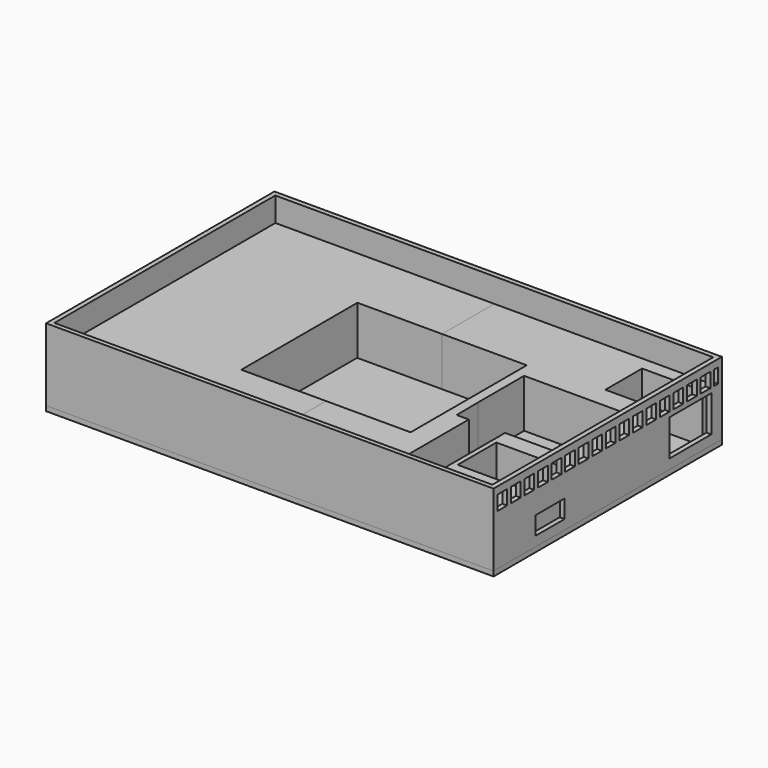
from build123d import *

# Parameters (mm, degrees)
F1_DEPTH = 2
F0_W     = 41
F0_H     = 23.8580039246
F0_W_2   = 35
F0_H_2   = 30
F0_W_3   = 14.5
F0_H_3   = 19
F0_W_4   = 10.5
F3_DEPTH = 22
F4_DEPTH = 30
F5_W     = 29.3693448901
F5_H     = 20
F6_DEPTH = 22
F7_W     = 5
F7_H     = 6
F7_W_2   = 2
F7_W_3   = 15
F7_H_2   = 7.5
F7_W_4   = 21.5
F7_H_3   = 15
F8_DEPTH = 2


with BuildPart() as f1:
    # F0 (on Top) → F1 (new body)
    with BuildSketch(Plane.XY):
        Polygon((29.8828537283, 118), (-155.1171462717, 118), (-155.1171462717, 0), (29.8828537283, 0), (29.8828537283, 47.8673752217), align=None)
        Polygon((27.8828537283, 108.5818558931), (27.8828537283, 47.8439224922), (27.8828537283, 9.4181441069), (27.8828537283, 2), (27.8251939824, 2), (27.8251939824, 1.8636477081), (-62.6748060176, 1.8636477081), (-153.1748060176, 1.8636477081), (-153.1748060176, 58.8636477081), (-153.1748060176, 115.8636477081), (-153.1171462717, 115.8636477081), (-153.1171462717, 116), (27.8828537283, 116), align=None, mode=Mode.SUBTRACT)
    extrude(amount=F1_DEPTH)


with BuildPart() as f1b:
    # F0 (on Top) → F1, piece 2 (new body)
    with BuildSketch(Plane.XY):
        Polygon((27.8251939824, 20.7216516327), (27.8251939824, 40.7216516327), (-1.5441509077, 40.7216516327), (-1.5441509077, 30.7216516327), (-1.5441509077, 20.7216516327), align=None)
    extrude(amount=F1_DEPTH)


with BuildPart() as f1c:
    # F0 (on Top) → F1, piece 3 (new body)
    with BuildSketch(Plane.XY):
        Polygon((-1.5441509077, 47.7216516327), (17.4558490923, 47.7216516327), (17.3251939824, 58.8636477081), (-23.6748060176, 58.8636477081), (-23.5441509077, 47.7216516327), (-18.5441509077, 47.7216516327), (-18.5441509077, 13.7216516327), (-3.5441509077, 13.7216516327), (-3.5441509077, 47.7216516327), align=None)
        with Locations((-3.1748060176, 70.7926496704)):
            Rectangle(F0_W, F0_H)
    extrude(amount=F1_DEPTH)


with BuildPart() as f1d:
    # F0 (on Top) → F1, piece 4 (new body)
    with BuildSketch(Plane.XY):
        with Locations((-45.1748060176, 73.8636477081)):
            Rectangle(F0_W_2, F0_H_2)
        with Locations((-80.1748060176, 73.8636477081)):
            Rectangle(F0_W_2, F0_H_2)
        with Locations((-80.1748060176, 43.8636477081)):
            Rectangle(F0_W_2, F0_H_2)
        with Locations((-45.1748060176, 43.8636477081)):
            Rectangle(F0_W_2, F0_H_2)
    extrude(amount=F1_DEPTH)


with BuildPart() as f1e:
    # F0 (on Top) → F1, piece 5 (new body)
    with BuildSketch(Plane.XY):
        with Locations((10.0751939824, 100.8636477081)):
            Rectangle(F0_W_3, F0_H_3)
        with Locations((22.5751939824, 100.8636477081)):
            Rectangle(F0_W_4, F0_H_3)
    extrude(amount=F1_DEPTH)


with BuildPart() as f3:
    # F2 (on Top) → F3 (new body)
    with BuildSketch(Plane.XY):
        Polygon((-62.6127840281, 116.0047547296), (-153.1127840281, 116.0047547296), (-153.1127840281, 59.0047547296), (-97.6127840281, 59.0047547296), (-97.6127840281, 89.0047547296), (-62.6127840281, 89.0047547296), align=None)
        Polygon((-97.6127840281, 59.0047547296), (-153.1127840281, 59.0047547296), (-153.1127840281, 2.0047547296), (-62.6127840281, 2.0047547296), (-62.6127840281, 29.0047547296), (-97.6127840281, 29.0047547296), align=None)
    extrude(amount=F3_DEPTH)


with BuildPart() as f4:
    # F4 (new): a face of the model
    f4_faces = [f1.part.faces().sort_by_distance(p)[0] for p in [
        (-62.6171462717, 117.7805711961, 2),
    ]]
    extrude(f4_faces, amount=F4_DEPTH)

    # F7 (on face) → F8 (cut)
    with BuildSketch(Plane.YZ.offset(29.8828537283)):
        with Locations((4.5, 26)):
            Rectangle(F7_W, F7_H)
        with Locations((11.5, 26)):
            Rectangle(F7_W, F7_H)
        with Locations((18.5, 26)):
            Rectangle(F7_W, F7_H)
        with Locations((25.5, 26)):
            Rectangle(F7_W, F7_H)
        with Locations((32.5, 26)):
            Rectangle(F7_W, F7_H)
        with Locations((39.5, 26)):
            Rectangle(F7_W, F7_H)
        with Locations((46.5, 26)):
            Rectangle(F7_W, F7_H)
        with Locations((53.5, 26)):
            Rectangle(F7_W, F7_H)
        with Locations((60.5, 26)):
            Rectangle(F7_W, F7_H)
        with Locations((67.5, 26)):
            Rectangle(F7_W, F7_H)
        with Locations((74.5, 26)):
            Rectangle(F7_W, F7_H)
        with Locations((81.5, 26)):
            Rectangle(F7_W, F7_H)
        with Locations((88.5, 26)):
            Rectangle(F7_W, F7_H)
        with Locations((95.5, 26)):
            Rectangle(F7_W, F7_H)
        with Locations((102.5, 26)):
            Rectangle(F7_W, F7_H)
        with Locations((109.5, 26)):
            Rectangle(F7_W, F7_H)
        with Locations((115, 26)):
            Rectangle(F7_W_2, F7_H)
        with Locations((29.22165, 9.75)):
            Rectangle(F7_W_3, F7_H_2)
        with Locations((101.75, 13.5)):
            Rectangle(F7_W_4, F7_H_3)
    extrude(amount=-F8_DEPTH, mode=Mode.SUBTRACT)


with BuildPart() as f6:
    # F5 (on face) → F6 (new body)
    with BuildSketch(Plane(origin=(0, 0, 0), x_dir=(1, 0, 0), z_dir=(0, 0, -1))):
        Polygon((-27.6127840281, -29.0047547296), (-27.6127840281, -59.0047547296), (-23.6748060176, -59.0047547296), (-23.6748060176, -58.8636477081), (-23.5441509077, -47.7216516327), (-18.5441509077, -47.7216516327), (-18.5441509077, -13.7216516327), (-3.5441509077, -13.7216516327), (-3.5441509077, -47.7216516327), (17.4558490923, -47.7216516327), (17.3251939824, -58.8636477081), (17.3251939824, -59.0047547296), (20.3872159719, -59.0047547296), (27.8828537283, -59.0047547296), (27.8828537283, -2), (27.8251939824, -2), (27.8251939824, -1.8636477081), (-62.6171462717, -1.8636477081), (-62.6161089932, -29.0047547296), (-62.6127840281, -29.0047547296), align=None)
        with Locations((13.1405215374, -30.7216516327)):
            Rectangle(F5_W, F5_H, mode=Mode.SUBTRACT)
        Polygon((-27.6127840281, -89.0047547296), (-62.6127840281, -89.0047547296), (-62.6127840281, -116), (27.8828537283, -116), (27.8828537283, -110.5047564595), (2.8828537283, -110.5047564595), (2.8828537283, -91.5047564595), (27.8828537283, -91.5047564595), (27.8828537283, -59.0047547296), (20.3872159719, -59.0047547296), (17.3251939824, -59.0047547296), (17.3251939824, -82.7216516327), (-23.6748060176, -82.7216516327), (-23.6748060176, -59.0047547296), (-27.6127840281, -59.0047547296), align=None)
    extrude(amount=-F6_DEPTH)


solid = Compound([f1.part, f1b.part, f1c.part, f1d.part, f1e.part, f3.part, f4.part, f6.part])
